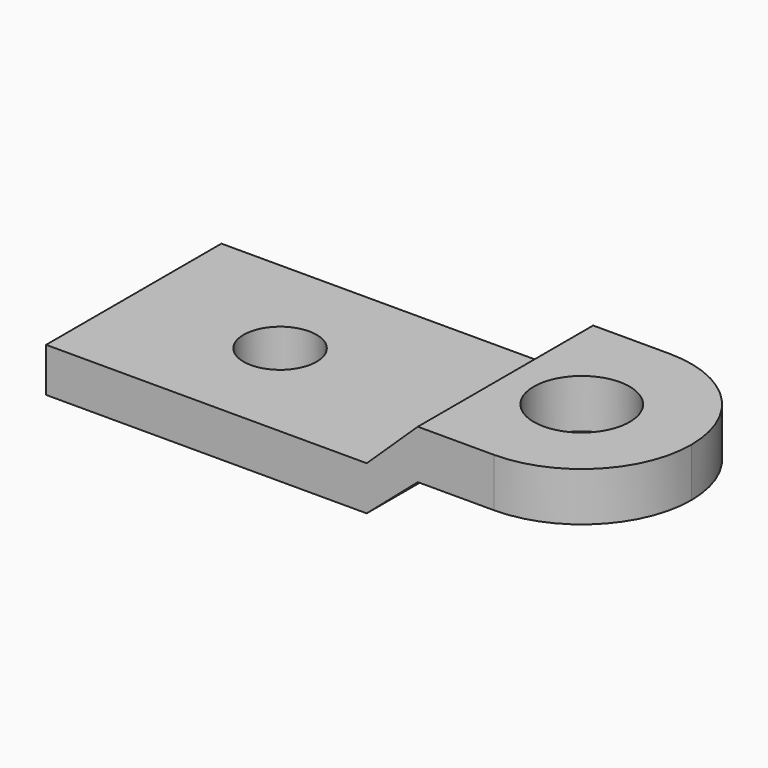
from build123d import *

# Parameters (mm, degrees)
F1_DEPTH = 12
F2_R     = 6
F3_R     = 5.99999
F5_D     = 5.25
F5_DEPTH = 12
F5_TIP   = 1.5772591249
F7_D     = 4
F7_DEPTH = 12
F7_TIP   = 1.2017212381


# Not quite as in the source:
# - a fillet or chamfer is up to 0.001 mm smaller than in the source, because OpenCascade refuses the exact size


with BuildPart() as f1:
    # F0 (on Front) → F1 (new body)
    with BuildSketch(Plane.XZ):
        Polygon((17.5538621843, 0), (0, 0), (0, -2.4168363307), (17.5538621843, -2.4168363307), (20.3523058444, 0), (30.528459698, 0), (30.528459698, 2.6712401304), (20.3523058444, 2.6712401304), align=None)
    extrude(amount=F1_DEPTH)

    # F2
    f2_edges = [f1.edges().sort_by_distance(p)[0] for p in [
        (30.52846, 0, 1.33562),
    ]]
    fillet(f2_edges, radius=F2_R)

    # F3 (radius 6 in the source; OpenCascade refuses exactly that, so slightly less here)
    f3_edges = [f1.edges().sort_by_distance(p)[0] for p in [
        (30.52846, -12, 1.33562),
    ]]
    fillet(f3_edges, radius=F3_R)

    # F5
    with Locations(Plane.XY.offset(2.6712401304)):
        with Locations((24.528459698, -6)):
            Hole(F5_D / 2, depth=F5_DEPTH)
            with Locations((0, 0, -(F5_DEPTH + F5_TIP / 2))):  # 118° drill point
                Cone(0, F5_D / 2, F5_TIP, mode=Mode.SUBTRACT)

    # F7
    with Locations(Plane.XY):
        with Locations((8.0127185211, -6)):
            Hole(F7_D / 2, depth=F7_DEPTH)
            with Locations((0, 0, -(F7_DEPTH + F7_TIP / 2))):  # 118° drill point
                Cone(0, F7_D / 2, F7_TIP, mode=Mode.SUBTRACT)


solid = f1.part
